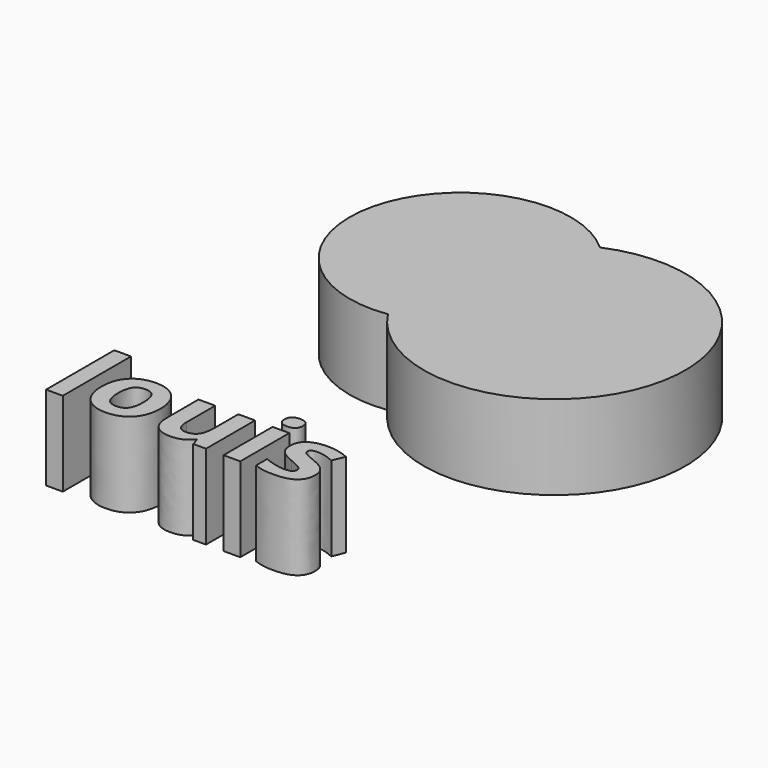
from build123d import *

# Parameters (mm, degrees)
F0_TEXT_SIZE = 16.8794766068
F1_DEPTH     = 12.7


# Not quite as in the source:
# - Text() gives the source's letters only with a copy of the font that has no kerning and outlines rounded to 1/6400 em; it was checked with that copy


with BuildPart() as f1:
    # F0 (on Top) → F1 (new body)
    with BuildSketch(Plane.XY):
        with BuildLine():
            ThreePointArc((-23.319407909, 2.0021655299), (-1.2286187107, -6.1583205041), (12.8645463786, 12.7090904862))
            ThreePointArc((12.8645463786, 12.7090904862), (4.054421285, 29.1127228818), (-14.4863436205, 30.8266355555))
            ThreePointArc((-14.4863436205, 30.8266355555), (-10.4273523581, 25.2338166725), (-8.9917467087, 18.4740778059))
            ThreePointArc((-8.9917467087, 18.4740778059), (-13.0748440114, 7.5584265484), (-23.319407909, 2.0021655299))
        make_face()
        with BuildLine():
            ThreePointArc((-8.9917467087, 18.4740778059), (-10.4273523581, 25.2338166725), (-14.4863436205, 30.8266355555))
            ThreePointArc((-14.4863436205, 30.8266355555), (-25.6241112947, 18.4740778059), (-23.319407909, 2.0021655299))
            ThreePointArc((-23.319407909, 2.0021655299), (-13.0748440114, 7.5584265484), (-8.9917467087, 18.4740778059))
        make_face()
        with BuildLine():
            ThreePointArc((-23.319407909, 2.0021655299), (-25.6241112947, 18.4740778059), (-14.4863436205, 30.8266355555))
            ThreePointArc((-14.4863436205, 30.8266355555), (-41.5265490046, 23.3472725085), (-23.319407909, 2.0021655299))
        make_face()
        with Locations((-44.0071634948, -38.0530357361)):
            Text('louis', F0_TEXT_SIZE, font='Open Sans', font_style=FontStyle.BOLD, text_align=(TextAlign.LEFT, TextAlign.BOTTOM))
    extrude(amount=F1_DEPTH)


solid = f1.part
